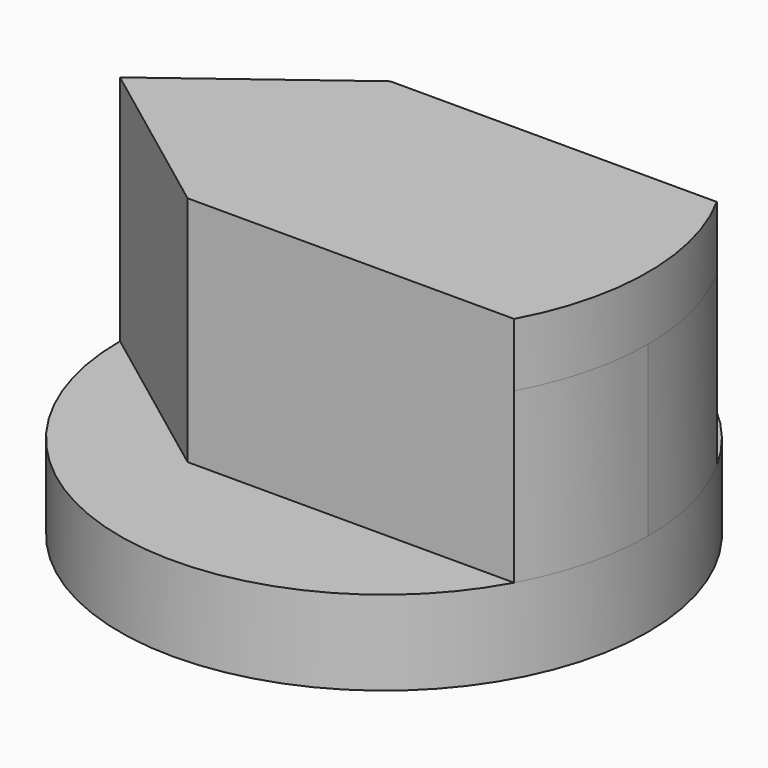
from build123d import *

# Parameters (mm, degrees)
F0_R     = 12.5
F1_DEPTH = 4
F2_R     = 0.5
F3_DEPTH = 8
F6_DEPTH = 3


# Not quite as in the source:
# - a fillet or chamfer that OpenCascade refuses, or shapes differently, is made with other operations: its cross-section is extruded or revolved along the edge and cut away or added


with BuildPart() as f1:
    # F0 (on Top) → F1 (new body)
    with BuildSketch(Plane.XY):
        Circle(F0_R)
        with BuildLine():
            Line((-2.2, -2.3237900077), (-2.2, 2.3237900077))
            ThreePointArc((-2.2, 2.3237900077), (3.2, 0), (-2.2, -2.3237900077))
        make_face(mode=Mode.SUBTRACT)
    extrude(amount=F1_DEPTH)

    # F2 (on face) → F3 (join)
    with BuildSketch(Plane.XY.offset(4)):
        with BuildLine():
            Line((-4.5, 6), (-12.5, 0))
            Line((-12.5, 0), (-4.5, -6))
            Line((-4.5, -6), (10.9658560997, -6))
            ThreePointArc((10.9658560997, -6), (12.1103922572, -3.0965140685), (12.5, 0))
            ThreePointArc((12.5, 0), (12.1103922572, 3.0965140685), (10.9658560997, 6))
            Line((10.9658560997, 6), (-4.5, 6))
        make_face()
        Circle(F2_R, mode=Mode.SUBTRACT)
    extrude(amount=F3_DEPTH)

    # F4: chamfer of 10 x 2.6794919243 on 1 edges, made by hand


with BuildPart() as f4_tool2:
    # F4_s3 → F4_t4 (revolve)
    with BuildSketch(Plane.XZ):
        Polygon((3.1794919243, 4), (0.5, 14), (0.5, 4), align=None)
    revolve(axis=Axis((0, 0, 4), (0, 0, 1)))

    split(bisect_by=Plane.YZ.offset(-2.2), keep=Keep.TOP)


with BuildPart() as f1_1:
    add(f1.part)

    # F4_t1: cut F4_tool2
    add(f4_tool2.part, mode=Mode.SUBTRACT)

    # F5 (on face) → F6 (join)
    with BuildSketch(Plane.XY.offset(12)):
        with BuildLine():
            Line((-4.5, 6), (-12.5, 0))
            Line((-12.5, 0), (-4.5, -6))
            Line((-4.5, -6), (10.9658560997, -6))
            ThreePointArc((10.9658560997, -6), (12.5, 0), (10.9658560997, 6))
            Line((10.9658560997, 6), (-4.5, 6))
        make_face()
    extrude(amount=F6_DEPTH)


solid = f1_1.part
